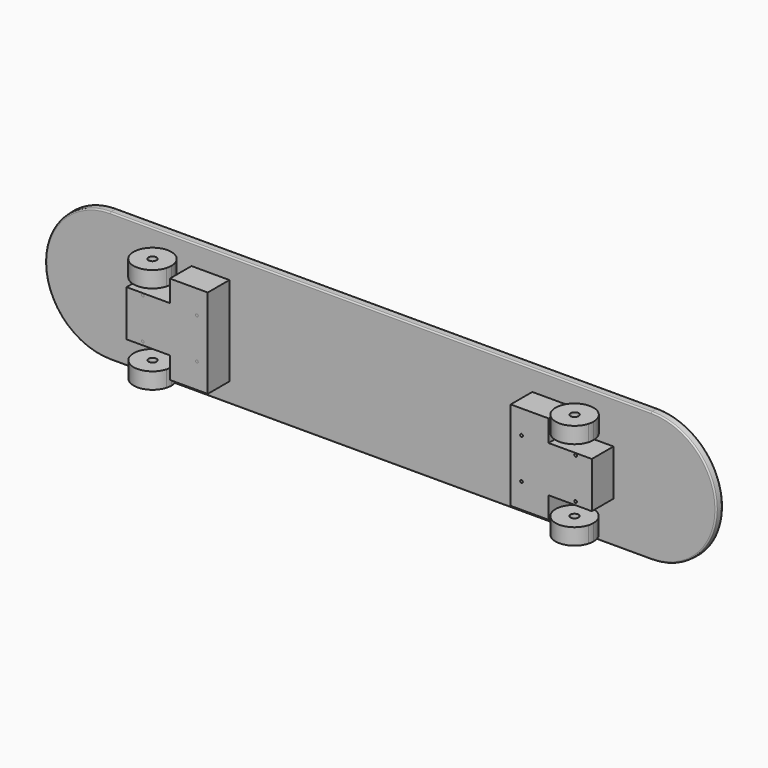
from build123d import *

# Parameters (mm, degrees)
F1_DEPTH  = 14
F1_TAPER  = -3
F3_R      = 2.5
F4_R      = 2.5
F6_DEPTH  = 50
F7_DEPTH  = 50
F2_R      = 2.5
F8_DEPTH  = 14.0010001
F10_R     = 2.5
F11_DEPTH = 70
F22_START = 25
F21_R     = 7.5
F22_DEPTH = 30
F24_START = 25
F23_R     = 7.5
F24_DEPTH = 30
F26_START = 25
F25_R     = 7.5
F26_DEPTH = 30
F28_START = 25
F27_R     = 7.5
F28_DEPTH = 30


# Not quite as in the source:
# - the program builds the solid bodies; features that only make, move or delete a surface that nothing else refers to are left out


with BuildPart() as f1:
    # F0 (on Front) → F1 (new body)
    with BuildSketch(Plane.XZ):
        with BuildLine():
            Line((-500, 0), (0, 0))
            Line((0, 0), (500, 0))
            ThreePointArc((500, 0), (620, 120), (500, 240))
            Line((500, 240), (-500, 240))
            ThreePointArc((-500, 240), (-620, 120), (-500, 0))
        make_face()
    extrude(amount=-F1_DEPTH, taper=F1_TAPER)

    # F3
    f3_edges = [f1.edges().sort_by_distance(p)[0] for p in [
        (-620, 0, 120),
    ]]
    fillet(f3_edges, radius=F3_R)

    # F4
    f4_edges = [f1.edges().sort_by_distance(p)[0] for p in [
        (620.733709, 14, 120),
    ]]
    fillet(f4_edges, radius=F4_R)

    # F2 (on face) → F8 (cut, through all)
    with BuildSketch(Plane.XZ):
        with Locations((-400, 157.5)):
            Circle(F2_R)
        with Locations((-300, 157.5)):
            Circle(F2_R)
        with Locations((-400, 82.5)):
            Circle(F2_R)
        with Locations((-300, 82.5)):
            Circle(F2_R)
        with Locations((400, 82.5)):
            Circle(F2_R)
        with Locations((300, 82.5)):
            Circle(F2_R)
        with Locations((300, 157.5)):
            Circle(F2_R)
        with Locations((400, 157.5)):
            Circle(F2_R)
    extrude(amount=-F8_DEPTH, mode=Mode.SUBTRACT)


with BuildPart() as f6:
    # F5 (on Front) → F6 (new body)
    with BuildSketch(Plane.XZ):
        Polygon((-350, 161.3137942916), (-430, 161.3137942916), (-430, 76.3137942916), (-350, 76.3137942916), (-350, 36.3137942916), (-280, 36.3137942916), (-280, 76.3137942916), (-280, 161.3137942916), (-280, 201.3137942916), (-350, 201.3137942916), align=None)
    extrude(amount=F6_DEPTH)


with BuildPart() as f7:
    # F5 (on Front) → F7 (new body)
    with BuildSketch(Plane.XZ):
        Polygon((-350, 161.3137942916), (-430, 161.3137942916), (-430, 76.3137942916), (-350, 76.3137942916), (-350, 36.3137942916), (-280, 36.3137942916), (-280, 76.3137942916), (-280, 161.3137942916), (-280, 201.3137942916), (-350, 201.3137942916), align=None)
    extrude(amount=F7_DEPTH)


with BuildPart() as f7b:
    # F5 (on Front) → F7, piece 2 (new body)
    with BuildSketch(Plane.XZ):
        Polygon((350, 161.3137942916), (350, 201.3137942916), (280, 201.3137942916), (280, 161.3137942916), (280, 76.3137942916), (280, 36.3137942916), (350, 36.3137942916), (350, 76.3137942916), (430, 76.3137942916), (430, 161.3137942916), align=None)
    extrude(amount=F7_DEPTH)


with BuildPart() as f11:
    # F10 (on face) → F11 (new body)
    with BuildSketch(Plane(origin=(0, 14, 0), x_dir=(-1, 0, 0), z_dir=(0, 1, 0))):
        with Locations((400, 82.5)):
            Circle(F10_R)
    extrude(amount=-F11_DEPTH)


with BuildPart() as f11b:
    # F10 (on face) → F11, piece 2 (new body)
    with BuildSketch(Plane(origin=(0, 14, 0), x_dir=(-1, 0, 0), z_dir=(0, 1, 0))):
        with Locations((400, 157.5)):
            Circle(F10_R)
    extrude(amount=-F11_DEPTH)


with BuildPart() as f11c:
    # F10 (on face) → F11, piece 3 (new body)
    with BuildSketch(Plane(origin=(0, 14, 0), x_dir=(-1, 0, 0), z_dir=(0, 1, 0))):
        with Locations((300, 82.5)):
            Circle(F10_R)
    extrude(amount=-F11_DEPTH)


with BuildPart() as f11d:
    # F10 (on face) → F11, piece 4 (new body)
    with BuildSketch(Plane(origin=(0, 14, 0), x_dir=(-1, 0, 0), z_dir=(0, 1, 0))):
        with Locations((300, 157.5)):
            Circle(F10_R)
    extrude(amount=-F11_DEPTH)


with BuildPart() as f11e:
    # F10 (on face) → F11, piece 5 (new body)
    with BuildSketch(Plane(origin=(0, 14, 0), x_dir=(-1, 0, 0), z_dir=(0, 1, 0))):
        with Locations((-300, 82.5)):
            Circle(F10_R)
    extrude(amount=-F11_DEPTH)


with BuildPart() as f11f:
    # F10 (on face) → F11, piece 6 (new body)
    with BuildSketch(Plane(origin=(0, 14, 0), x_dir=(-1, 0, 0), z_dir=(0, 1, 0))):
        with Locations((-300, 157.5)):
            Circle(F10_R)
    extrude(amount=-F11_DEPTH)


with BuildPart() as f11g:
    # F10 (on face) → F11, piece 7 (new body)
    with BuildSketch(Plane(origin=(0, 14, 0), x_dir=(-1, 0, 0), z_dir=(0, 1, 0))):
        with Locations((-400, 82.5)):
            Circle(F10_R)
    extrude(amount=-F11_DEPTH)


with BuildPart() as f11h:
    # F10 (on face) → F11, piece 8 (new body)
    with BuildSketch(Plane(origin=(0, 14, 0), x_dir=(-1, 0, 0), z_dir=(0, 1, 0))):
        with Locations((-400, 157.5)):
            Circle(F10_R)
    extrude(amount=-F11_DEPTH)


with BuildPart() as f7b_1:
    add(f7b.part)

    # F12: cut F11d, F11c, F11, F11b, F11e, F11f, F11h, F11g
    add(f11d.part, mode=Mode.SUBTRACT)
    add(f11c.part, mode=Mode.SUBTRACT)
    add(f11.part, mode=Mode.SUBTRACT)
    add(f11b.part, mode=Mode.SUBTRACT)
    add(f11e.part, mode=Mode.SUBTRACT)
    add(f11f.part, mode=Mode.SUBTRACT)
    add(f11h.part, mode=Mode.SUBTRACT)
    add(f11g.part, mode=Mode.SUBTRACT)


with BuildPart() as f7_1:
    add(f7.part)

    # F12: cut F11d, F11c, F11, F11b, F11e, F11f, F11h, F11g
    add(f11d.part, mode=Mode.SUBTRACT)
    add(f11c.part, mode=Mode.SUBTRACT)
    add(f11.part, mode=Mode.SUBTRACT)
    add(f11b.part, mode=Mode.SUBTRACT)
    add(f11e.part, mode=Mode.SUBTRACT)
    add(f11f.part, mode=Mode.SUBTRACT)
    add(f11h.part, mode=Mode.SUBTRACT)
    add(f11g.part, mode=Mode.SUBTRACT)


with BuildPart() as f22:
    # F21 (on face) → F22 (new body)
    with BuildSketch(Plane.XY.offset(161.3137942916).offset(F22_START)):
        with BuildLine():
            ThreePointArc((423.4911083874, -50), (424.6207220719, -44.9727315677), (425, -39.8340933025))
            ThreePointArc((425, -39.8340933025), (384.8613617348, -5.2133712306), (356.5088916126, -50))
            Line((356.5088916126, -50), (423.4911083874, -50))
        make_face()
        with Locations((390, -39.8340933025)):
            Circle(F21_R, mode=Mode.SUBTRACT)
        with BuildLine():
            Line((423.4911083874, -50), (356.5088916126, -50))
            ThreePointArc((356.5088916126, -50), (390, -74.8340933025), (423.4911083874, -50))
        make_face()
    extrude(amount=F22_DEPTH)


with BuildPart() as f24:
    # F23 (on face) → F24 (new body)
    with BuildSketch(Plane(origin=(0, 0, 76.3137942916), x_dir=(1, 0, 0), z_dir=(0, 0, -1)).offset(F24_START)):
        with BuildLine():
            ThreePointArc((356.4589803375, 50), (384.9470646248, 5.3666657093), (425, 40))
            ThreePointArc((425, 40), (424.6333342907, 45.0529353752), (423.5410196625, 50))
            Line((423.5410196625, 50), (356.4589803375, 50))
        make_face()
        with Locations((390, 40)):
            Circle(F23_R, mode=Mode.SUBTRACT)
        with BuildLine():
            Line((356.4589803375, 50), (423.5410196625, 50))
            ThreePointArc((423.5410196625, 50), (390, 75), (356.4589803375, 50))
        make_face()
    extrude(amount=F24_DEPTH)


with BuildPart() as f26:
    # F25 (on face) → F26 (new body)
    with BuildSketch(Plane.XY.offset(161.3137942916).offset(F26_START)):
        with BuildLine():
            Line((-356.3969283225, -50), (-423.6030716775, -50))
            ThreePointArc((-423.6030716775, -50), (-390, -75.2105376124), (-356.3969283225, -50))
        make_face()
        with BuildLine():
            ThreePointArc((-356.3969283225, -50), (-355.3509920148, -45.1548520891), (-355, -40.2105376124))
            ThreePointArc((-355, -40.2105376124), (-394.9443144766, -5.5615296273), (-423.6030716775, -50))
            Line((-423.6030716775, -50), (-356.3969283225, -50))
        make_face()
        with Locations((-390, -40.2105376124)):
            Circle(F25_R, mode=Mode.SUBTRACT)
    extrude(amount=F26_DEPTH)


with BuildPart() as f28:
    # F27 (on face) → F28 (new body)
    with BuildSketch(Plane(origin=(0, 0, 76.3137942916), x_dir=(1, 0, 0), z_dir=(0, 0, -1)).offset(F28_START)):
        with BuildLine():
            Line((-423.5410196625, 50), (-356.4589803375, 50))
            ThreePointArc((-356.4589803375, 50), (-390, 75), (-423.5410196625, 50))
        make_face()
        with BuildLine():
            ThreePointArc((-423.5410196625, 50), (-395.0529353752, 5.3666657093), (-355, 40))
            ThreePointArc((-355, 40), (-355.3666657093, 45.0529353752), (-356.4589803375, 50))
            Line((-356.4589803375, 50), (-423.5410196625, 50))
        make_face()
        with Locations((-390, 40)):
            Circle(F27_R, mode=Mode.SUBTRACT)
    extrude(amount=F28_DEPTH)


solid = Compound([f1.part, f6.part, f7b_1.part, f7_1.part, f22.part, f24.part, f26.part, f28.part])
